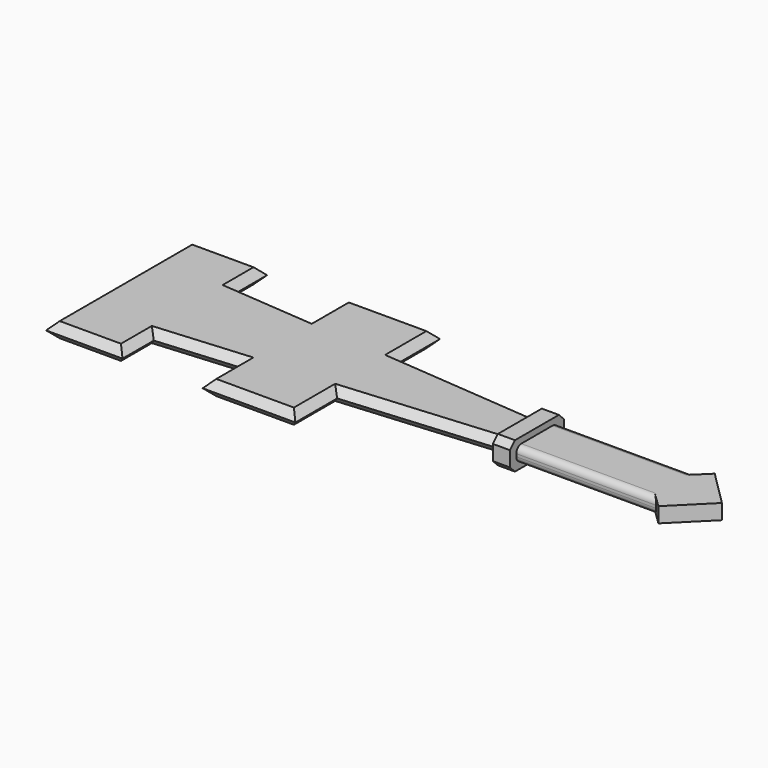
from build123d import *

# Parameters (mm, degrees)
F2_DEPTH = 4.318
F3_SIZE  = 2.15899
F5_DEPTH = 1.778
F7_DEPTH = 1.778
F8_R     = 1.778
F9_SIZE  = 1.778


# Not quite as in the source:
# - a fillet or chamfer is up to 0.001 mm smaller than in the source, because OpenCascade refuses the exact size


with BuildPart() as f2:
    # F0 (on Top) → F2 (new body)
    with BuildSketch(Plane.XY):
        Polygon((27.5745280087, 3.6292271689), (27.5745280087, 1.2858584523), (27.5745280087, -13.2207097486), (27.5745280087, -15.5640784651), (32.4286483228, -15.5640784651), (32.4286483228, -13.3150536567), (32.4286483228, 1.3802023605), (32.4286483228, 3.6292271689), align=None)
        Polygon((72.2789242864, 1.3802023605), (32.4286483228, 1.3802023605), (32.4286483228, -13.3150536567), (72.2789242864, -13.3150536567), (75.0406160951, -15.9978345037), (85.1087123156, -5.9674256481), (75.0406160951, 4.0629832074), align=None)
        Polygon((-64.9878308177, 19.7724616155), (-86.7510214448, 19.7724616155), (-86.7510214448, -31.7073129117), (-64.9878308177, -31.7073129117), (-64.9878308177, -20.5603092909), (-42.1630144119, -18.7024753541), (-42.1630144119, -31.7073129117), (-15.7552305609, -31.7073129117), (-15.7552305609, -16.8446414173), (27.5745280087, -13.2207097486), (27.5745280087, 1.2858584523), (-15.7552305609, 4.909790121), (-15.7552305609, 19.7724616155), (-42.1630144119, 19.7724616155), (-42.1630144119, 6.7676240578), (-64.9878308177, 8.6254579946), align=None)
    extrude(amount=F2_DEPTH)

    # F3 (size 2.159 in the source; OpenCascade refuses exactly that, so slightly less here)
    f3_edges = [f2.edges().sort_by_distance(p)[0] for p in [
        (-53.575423, -19.631392, 4.318),
        (-42.163014, -25.204894, 4.318),
        (-28.959122, -31.707313, 4.318),
        (-15.755231, -24.275977, 4.318),
        (5.909649, -15.032676, 4.318),
        (5.909649, 3.097824, 4.318),
        (-15.755231, 12.341126, 4.318),
        (-28.959122, 19.772462, 4.318),
        (-42.163014, 13.270043, 4.318),
        (-53.575423, 7.696541, 4.318),
        (-64.987831, 14.19896, 4.318),
        (-75.869426, 19.772462, 4.318),
        (-86.751021, -5.967426, 4.318),
        (-75.869426, -31.707313, 4.318),
        (-64.987831, -26.133811, 4.318),
        (-28.959122, -31.707313, 0),
        (-15.755231, -24.275977, 0),
        (5.909649, -15.032676, 0),
        (-42.163014, -25.204894, 0),
        (-53.575423, -19.631392, 0),
        (-75.869426, -31.707313, 0),
        (-64.987831, -26.133811, 0),
        (-86.751021, -5.967426, 0),
        (-75.869426, 19.772462, 0),
        (-64.987831, 14.19896, 0),
        (-53.575423, 7.696541, 0),
        (-15.755231, 12.341126, 0),
        (5.909649, 3.097824, 0),
        (-42.163014, 13.270043, 0),
        (-28.959122, 19.772462, 0),
    ]]
    chamfer(f3_edges, length=F3_SIZE)

    # F4 (on face) → F5 (join)
    with BuildSketch(Plane.XY.offset(4.318)):
        Polygon((32.4286483228, 3.6292271689), (27.5745280087, 3.6292271689), (27.5745280087, 1.2858584523), (27.5745280087, -0.8806694518), (27.5745280087, -11.0541818444), (27.5745280087, -13.2207097486), (27.5745280087, -15.5640784651), (32.4286483228, -15.5640784651), (32.4286483228, -13.3150536567), (32.4286483228, 1.3802023605), align=None)
    extrude(amount=F5_DEPTH)

    # F6 (on face) → F7 (join)
    with BuildSketch(Plane(origin=(0, 0, 0), x_dir=(1, 0, 0), z_dir=(0, 0, -1))):
        Polygon((32.4286483228, 15.5640784651), (27.5745280087, 15.5640784651), (27.5745280087, 11.0541818444), (27.5745280087, 0.8806694518), (27.5745280087, -3.6292271689), (32.4286483228, -3.6292271689), (32.4286483228, -1.3802023605), (32.4286483228, 13.3150536567), align=None)
    extrude(amount=F7_DEPTH)

    # F8
    f8_edges = [f2.edges().sort_by_distance(p)[0] for p in [
        (52.353786, 1.380202, 0),
        (52.353786, -13.315054, 0),
        (52.353786, 1.380202, 4.318),
        (52.353786, -13.315054, 4.318),
    ]]
    fillet(f8_edges, radius=F8_R)

    # F9
    f9_edges = [f2.edges().sort_by_distance(p)[0] for p in [
        (30.001588, -15.564078, -1.778),
        (30.001588, -15.564078, 6.096),
        (30.001588, 3.629227, 6.096),
        (30.001588, 3.629227, -1.778),
    ]]
    chamfer(f9_edges, length=F9_SIZE)


solid = f2.part
